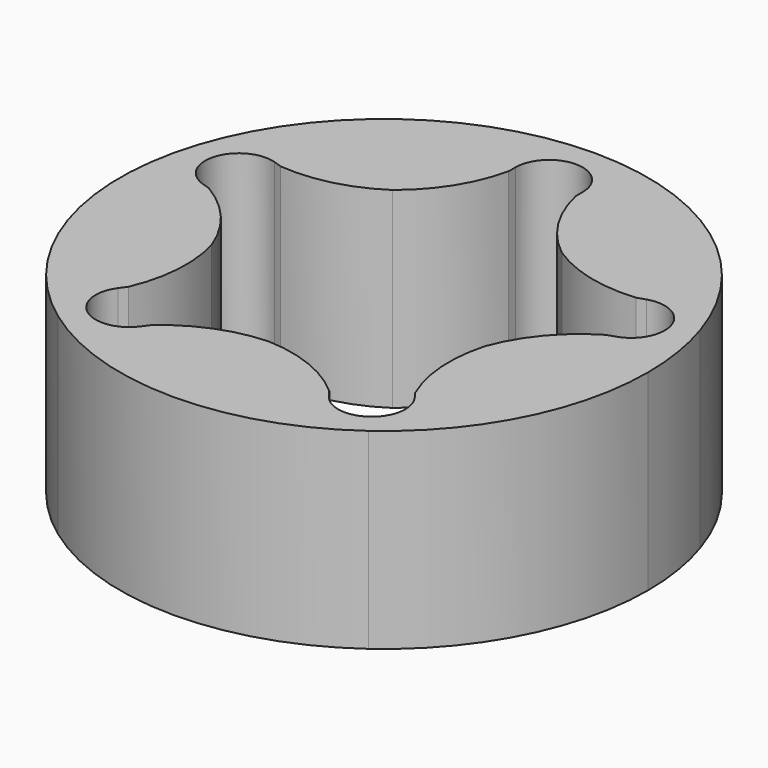
from build123d import *

# Parameters (mm, degrees)
F2_DEPTH = 25
F3_DEPTH = 20
F4_DEPTH = 25


with BuildPart() as f2:
    # F1 (on Top) → F2 (new body)
    with BuildSketch(Plane.XY):
        with BuildLine():
            ThreePointArc((-8.8167787844, 7.1352549156), (-13.4599944512, 5.0779075669), (-18.5244405716, 4.6990733883))
            Line((-18.5244405716, 4.6990733883), (-19.36615562, 4.9725631861))
            ThreePointArc((-19.36615562, 4.9725631861), (-23.7764129074, 2.7254248594), (-21.5292745807, -1.684832428))
            Line((-21.5292745807, -1.684832428), (-20.6875595323, -1.9583222258))
            ThreePointArc((-20.6875595323, -1.9583222258), (-16.813009697, -5.241612255), (-14.2658477444, -9.6352549156))
            ThreePointArc((-14.2658477444, -9.6352549156), (-13.7440266917, -14.6869707262), (-14.9487338959, -19.6206114097))
            Line((-14.9487338959, -19.6206114097), (-15.4689424046, -20.336616996))
            ThreePointArc((-15.4689424046, -20.336616996), (-14.6946313073, -25.2254248594), (-9.805823444, -24.4511137621))
            Line((-9.805823444, -24.4511137621), (-9.2856149352, -23.7351081758))
            ThreePointArc((-9.2856149352, -23.7351081758), (-4.9657188134, -21.0647847237), (0, -20))
            ThreePointArc((0, -20), (4.9657188134, -21.0647847237), (9.2856149352, -23.7351081758))
            Line((9.2856149352, -23.7351081758), (9.805823444, -24.4511137621))
            ThreePointArc((9.805823444, -24.4511137621), (14.6946313073, -25.2254248594), (15.4689424046, -20.336616996))
            Line((15.4689424046, -20.336616996), (14.9487338959, -19.6206114097))
            ThreePointArc((14.9487338959, -19.6206114097), (13.7440266917, -14.6869707262), (14.2658477444, -9.6352549156))
            ThreePointArc((14.2658477444, -9.6352549156), (16.813009697, -5.241612255), (20.6875595323, -1.9583222258))
            Line((20.6875595323, -1.9583222258), (21.5292745807, -1.684832428))
            ThreePointArc((21.5292745807, -1.684832428), (23.7764129074, 2.7254248594), (19.36615562, 4.9725631861))
            Line((19.36615562, 4.9725631861), (18.5244405716, 4.6990733883))
            ThreePointArc((18.5244405716, 4.6990733883), (13.4599944512, 5.0779075669), (8.8167787844, 7.1352549156))
            ThreePointArc((8.8167787844, 7.1352549156), (5.4252926325, 10.915460138), (3.5, 15.614968423))
            Line((3.5, 15.614968423), (3.5, 16.5))
            ThreePointArc((3.5, 16.5), (0, 20), (-3.5, 16.5))
            Line((-3.5, 16.5), (-3.5, 15.614968423))
            ThreePointArc((-3.5, 15.614968423), (-5.4252926325, 10.915460138), (-8.8167787844, 7.1352549156))
        make_face()
    extrude(amount=F2_DEPTH)

    # F0 (on Top) → F3 (join)
    with BuildSketch(Plane.XY):
        with BuildLine():
            ThreePointArc((16.164094438, -27.2479673453), (24.5026794152, -17.4847387428), (27.5, -5))
            ThreePointArc((27.5, -5), (27.1614293664, -0.6980522114), (26.1540541981, 3.4979673453))
            Line((26.1540541981, 3.4979673453), (23.7764129074, 2.7254248594))
            Line((23.7764129074, 2.7254248594), (0, -5))
            Line((0, -5), (14.6946313073, -25.2254248594))
            Line((14.6946313073, -25.2254248594), (16.164094438, -27.2479673453))
        make_face()
        with BuildLine():
            Line((23.7764129074, 2.7254248594), (26.1540541981, 3.4979673453))
            ThreePointArc((26.1540541981, 3.4979673453), (0, 22.5), (-26.1540541981, 3.4979673453))
            Line((-26.1540541981, 3.4979673453), (-23.7764129074, 2.7254248594))
            Line((-23.7764129074, 2.7254248594), (0, -5))
            Line((0, -5), (23.7764129074, 2.7254248594))
        make_face()
        with BuildLine():
            ThreePointArc((-16.164094438, -27.2479673453), (0, -32.5), (16.164094438, -27.2479673453))
            Line((16.164094438, -27.2479673453), (14.6946313073, -25.2254248594))
            Line((14.6946313073, -25.2254248594), (0, -5))
            Line((0, -5), (-14.6946313073, -25.2254248594))
            Line((-14.6946313073, -25.2254248594), (-16.164094438, -27.2479673453))
        make_face()
        with BuildLine():
            Line((-23.7764129074, 2.7254248594), (-26.1540541981, 3.4979673453))
            ThreePointArc((-26.1540541981, 3.4979673453), (-26.1540541981, -13.4979673453), (-16.164094438, -27.2479673453))
            Line((-16.164094438, -27.2479673453), (-14.6946313073, -25.2254248594))
            Line((-14.6946313073, -25.2254248594), (0, -5))
            Line((0, -5), (-23.7764129074, 2.7254248594))
        make_face()
    extrude(amount=F3_DEPTH)

    # F4 (cut): a face of the model
    f4_faces = [f2.faces().sort_by_distance(p)[0] for p in [
        (0, -5, 25),
    ]]
    extrude(f4_faces, amount=-F4_DEPTH, mode=Mode.SUBTRACT)


solid = f2.part
